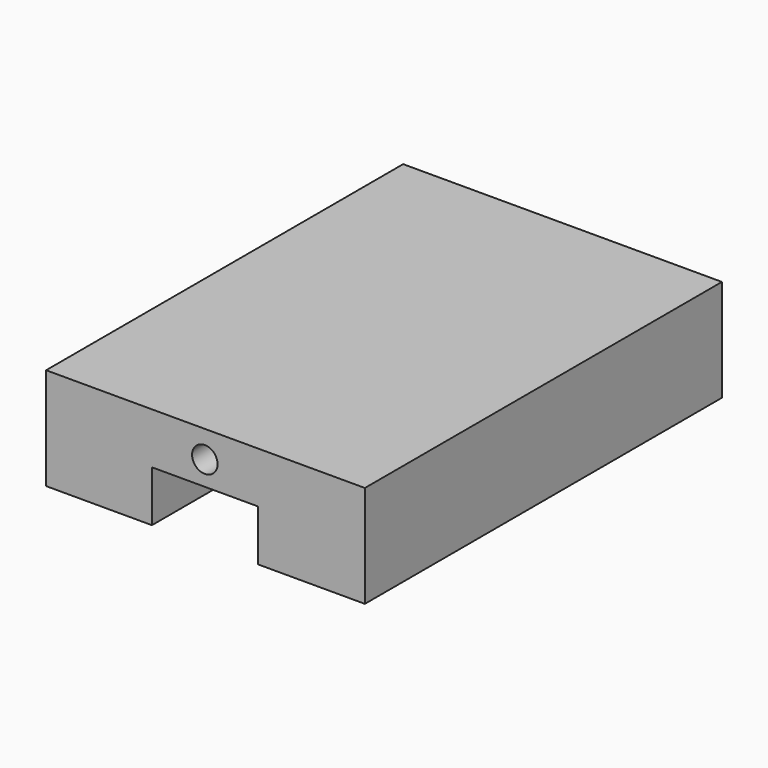
from build123d import *

# Parameters (mm, degrees)
F0_W     = 21.082
F0_H     = 88.9
F0_W_2   = 21.336
F1_DEPTH = 20.32
F2_DEPTH = 10.16
F3_R     = 2.54
F5_DEPTH = 88.9


# Not quite as in the source:
# - the program builds the solid bodies; features that only make, move or delete a surface that nothing else refers to are left out


with BuildPart() as f1:
    # F0 (on Top) → F1 (new body)
    with BuildSketch(Plane.XY):
        with Locations((-23.6977891486, 3.6070292577)):
            Rectangle(F0_W, F0_H)
        with Locations((-2.6157891486, 3.6070292577)):
            Rectangle(F0_W, F0_H)
        with Locations((18.5932108514, 3.6070292577)):
            Rectangle(F0_W_2, F0_H)
    extrude(amount=F1_DEPTH)

    # F0 (on Top) → F2 (cut)
    with BuildSketch(Plane.XY):
        with Locations((-2.6157891486, 3.6070292577)):
            Rectangle(F0_W, F0_H)
    extrude(amount=F2_DEPTH, mode=Mode.SUBTRACT)

    # F3 (on face) → F5 (cut)
    with BuildSketch(Plane(origin=(0, 48.0570292577, 0), x_dir=(-1, 0, 0), z_dir=(0, 1, 0))):
        with Locations((2.6157891486, 14.9523410946)):
            Circle(F3_R)
    extrude(amount=-F5_DEPTH, mode=Mode.SUBTRACT)


solid = f1.part
